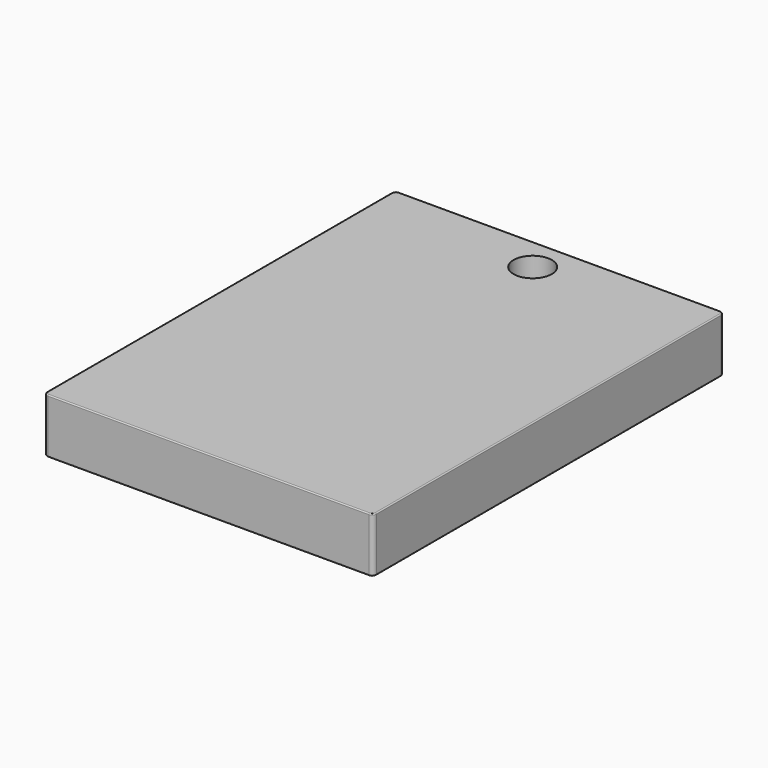
from build123d import *

# Parameters (mm, degrees)
F0_W         = 1524
F0_H         = 2032
F0_R         = 88.6274236121
F1_DEPTH     = 254
F2_R         = 5.08
F3_T1_DEPTH  = 254
F3_T4_ANGLE  = 90
F3_T6_ANGLE  = 90
F3_T8_ANGLE  = 90
F3_T10_ANGLE = 90
F3_T12_ANGLE = 90
F3_T14_ANGLE = 90
F3_T16_ANGLE = 90
F3_T18_ANGLE = 90


# Not quite as in the source:
# - a fillet or chamfer that OpenCascade refuses, or shapes differently, is made with other operations: its cross-section is extruded or revolved along the edge and cut away or added


with BuildPart() as f1:
    # F0 (on Top) → F1 (new body)
    with BuildSketch(Plane.XY):
        Rectangle(F0_W, F0_H)
        with Locations((0, 860.7016801834)):
            Circle(F0_R, mode=Mode.SUBTRACT)
    extrude(amount=F1_DEPTH)

    # F2
    f2_edges = [f1.edges().sort_by_distance(p)[0] for p in [
        (-762, 0, 254),
        (0, -1016, 254),
        (762, 0, 254),
        (0, 1016, 254),
        (0, 1016, 0),
        (762, 0, 0),
        (0, -1016, 0),
        (-762, 0, 0),
    ]]
    fillet(f2_edges, radius=F2_R)

    # F3: fillet of radius 19.05 on 4 edges, made by hand

    # F3_s2 → F3_t1 (cut)
    with BuildSketch(Plane.XY):
        with BuildLine():
            ThreePointArc((762, 996.95), (756.4203841816, 1010.4203841816), (742.95, 1016))
            Line((742.95, 1016), (762, 1016))
            Line((762, 1016), (762, 996.95))
        make_face()
        with BuildLine():
            ThreePointArc((762, -996.95), (756.4203841816, -1010.4203841816), (742.95, -1016))
            Line((742.95, -1016), (762, -1016))
            Line((762, -1016), (762, -996.95))
        make_face()
        with BuildLine():
            ThreePointArc((-742.95, -1016), (-756.4203841816, -1010.4203841816), (-762, -996.95))
            Line((-762, -996.95), (-762, -1016))
            Line((-762, -1016), (-742.95, -1016))
        make_face()
        with BuildLine():
            ThreePointArc((-742.95, 1016), (-756.4203841816, 1010.4203841816), (-762, 996.95))
            Line((-762, 996.95), (-762, 1016))
            Line((-762, 1016), (-742.95, 1016))
        make_face()
    extrude(amount=F3_T1_DEPTH, mode=Mode.SUBTRACT)

    # F3_s3 → F3_t4 (revolve, cut)
    with BuildSketch(Plane.XZ.offset(-996.95)):
        with BuildLine():
            ThreePointArc((-756.92, 0), (-760.5121024484, 1.4878975516), (-762, 5.08))
            Line((-762, 5.08), (-762, 0))
            Line((-762, 0), (-756.92, 0))
        make_face()
    revolve(axis=Axis((-742.95, 996.95, 0), (0, 0, -1)), revolution_arc=F3_T4_ANGLE, mode=Mode.SUBTRACT)

    # F3_s5 → F3_t6 (revolve, cut)
    with BuildSketch(Plane.YZ.offset(-742.95)):
        with BuildLine():
            ThreePointArc((1010.92, 254), (1014.5121024484, 252.5121024484), (1016, 248.92))
            Line((1016, 248.92), (1016, 254))
            Line((1016, 254), (1010.92, 254))
        make_face()
    revolve(axis=Axis((-742.95, 996.95, 254), (0, 0, 1)), revolution_arc=F3_T6_ANGLE, mode=Mode.SUBTRACT)

    # F3_s7 → F3_t8 (revolve, cut)
    with BuildSketch(Plane.YZ.offset(-742.95)):
        with BuildLine():
            ThreePointArc((-1010.92, 0), (-1014.5121024484, 1.4878975516), (-1016, 5.08))
            Line((-1016, 5.08), (-1016, 0))
            Line((-1016, 0), (-1010.92, 0))
        make_face()
    revolve(axis=Axis((-742.95, -996.95, 0), (0, 0, -1)), revolution_arc=F3_T8_ANGLE, mode=Mode.SUBTRACT)

    # F3_s9 → F3_t10 (revolve, cut)
    with BuildSketch(Plane.XZ.offset(996.95)):
        with BuildLine():
            ThreePointArc((-756.92, 254), (-760.5121024484, 252.5121024484), (-762, 248.92))
            Line((-762, 248.92), (-762, 254))
            Line((-762, 254), (-756.92, 254))
        make_face()
    revolve(axis=Axis((-742.95, -996.95, 254), (0, 0, 1)), revolution_arc=F3_T10_ANGLE, mode=Mode.SUBTRACT)

    # F3_s11 → F3_t12 (revolve, cut)
    with BuildSketch(Plane.XZ.offset(996.95)):
        with BuildLine():
            ThreePointArc((756.92, 0), (760.5121024484, 1.4878975516), (762, 5.08))
            Line((762, 5.08), (762, 0))
            Line((762, 0), (756.92, 0))
        make_face()
    revolve(axis=Axis((742.95, -996.95, 0), (0, 0, -1)), revolution_arc=F3_T12_ANGLE, mode=Mode.SUBTRACT)

    # F3_s13 → F3_t14 (revolve, cut)
    with BuildSketch(Plane.YZ.offset(742.95)):
        with BuildLine():
            ThreePointArc((-1010.92, 254), (-1014.5121024484, 252.5121024484), (-1016, 248.92))
            Line((-1016, 248.92), (-1016, 254))
            Line((-1016, 254), (-1010.92, 254))
        make_face()
    revolve(axis=Axis((742.95, -996.95, 254), (0, 0, 1)), revolution_arc=F3_T14_ANGLE, mode=Mode.SUBTRACT)

    # F3_s15 → F3_t16 (revolve, cut)
    with BuildSketch(Plane.YZ.offset(742.95)):
        with BuildLine():
            ThreePointArc((1010.92, 0), (1014.5121024484, 1.4878975516), (1016, 5.08))
            Line((1016, 5.08), (1016, 0))
            Line((1016, 0), (1010.92, 0))
        make_face()
    revolve(axis=Axis((742.95, 996.95, 0), (0, 0, -1)), revolution_arc=F3_T16_ANGLE, mode=Mode.SUBTRACT)

    # F3_s17 → F3_t18 (revolve, cut)
    with BuildSketch(Plane.XZ.offset(-996.95)):
        with BuildLine():
            ThreePointArc((756.92, 254), (760.5121024484, 252.5121024484), (762, 248.92))
            Line((762, 248.92), (762, 254))
            Line((762, 254), (756.92, 254))
        make_face()
    revolve(axis=Axis((742.95, 996.95, 254), (0, 0, 1)), revolution_arc=F3_T18_ANGLE, mode=Mode.SUBTRACT)


solid = f1.part
